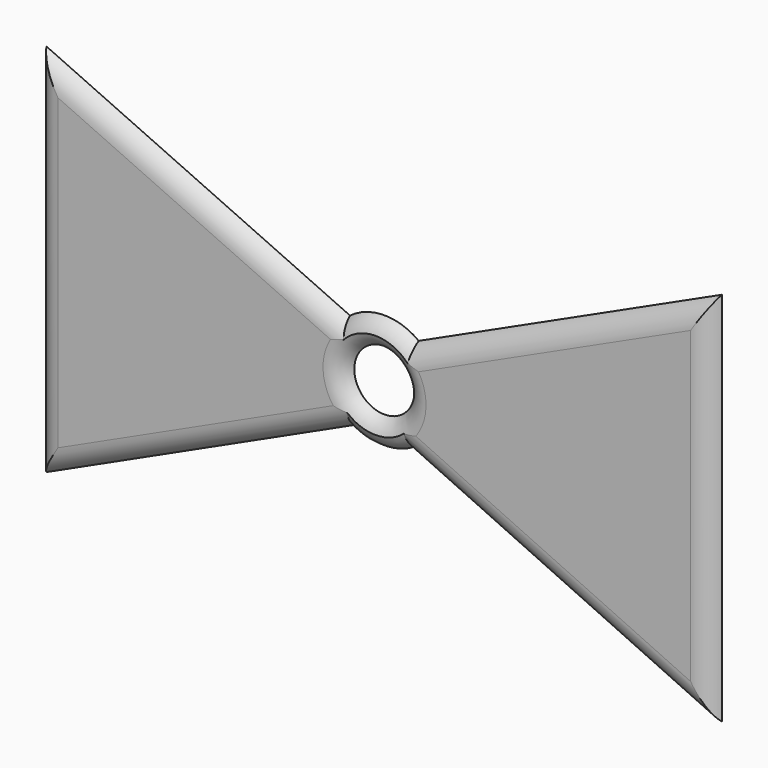
from build123d import *

# Parameters (mm, degrees)
F1_DEPTH     = 2.54
F2_T1_DEPTH  = 99.1010776341
F2_T3_DEPTH  = 99.3158813996
F2_T8_DEPTH  = 90.6208911446
F2_S9_R      = 11.7840069811
F2_T10_DEPTH = 49
F2_T14_DEPTH = 91.7966915257
F2_S15_R     = 11.7840069811
F2_T16_DEPTH = 49
F2_T20_ANGLE = 169.5184876271
F2_T26_ANGLE = 180.7013968541
F2_T32_DEPTH = 90.6339735213
F2_S33_R     = 11.7840069811
F2_T34_DEPTH = 49
F2_T38_DEPTH = 91.7098992775
F2_S39_R     = 11.7840069811
F2_T40_DEPTH = 49
F2_T47_DEPTH = 90.6208911446
F2_S48_R     = 11.7840069811
F2_T49_DEPTH = 49
F2_T52_ANGLE = 180.7013968541
F2_T60_DEPTH = 91.7966915257
F2_S61_R     = 11.7840069811
F2_T62_DEPTH = 49
F2_T65_ANGLE = 169.5184876271
F2_T73_ANGLE = 169.5184876271
F2_T78_DEPTH = 91.7098992775
F2_S79_R     = 11.7840069811
F2_T80_DEPTH = 49
F2_T86_DEPTH = 90.6339735213
F2_S87_R     = 11.7840069811
F2_T88_DEPTH = 49
F2_T91_ANGLE = 180.7013968541


# Not quite as in the source:
# - a fillet or chamfer that OpenCascade refuses, or shapes differently, is made with other operations: its cross-section is extruded or revolved along the edge and cut away or added


with BuildPart() as f1:
    # F0 (on Front) → F1 (new body)
    with BuildSketch(Plane.XZ):
        with BuildLine():
            Line((-31.3936966788, 53.9309575686), (-93.8453510125, 82.3742888697))
            Line((-93.8453510125, 82.3742888697), (-93.8453510125, 5.2702564917))
            Line((-93.8453510125, 5.2702564917), (-30.4330390113, 34.4399206311))
            ThreePointArc((-30.4330390113, 34.4399206311), (-36.0837561517, 43.9306053941), (-31.3936966788, 53.9309575686))
        make_face()
        with BuildLine():
            Line((-24.3140361377, 37.2546620127), (-30.4330390113, 34.4399206311))
            ThreePointArc((-30.4330390113, 34.4399206311), (-24.3162174043, 32.7266945746), (-18.1987619666, 34.4376560178))
            Line((-18.1987619666, 34.4376560178), (-24.3140361377, 37.2546620127))
        make_face()
        with BuildLine():
            ThreePointArc((-17.2562665131, 53.9473696458), (-24.3277161277, 56.2947003943), (-31.3936966788, 53.9309575686))
            Line((-31.3936966788, 53.9309575686), (-24.3140361377, 50.7065573118))
            Line((-24.3140361377, 50.7065573118), (-17.2562665131, 53.9473696458))
        make_face()
        with BuildLine():
            Line((-24.3140361377, 50.7065573118), (-31.3936966788, 53.9309575686))
            ThreePointArc((-31.3936966788, 53.9309575686), (-36.0837561517, 43.9306053941), (-30.4330390113, 34.4399206311))
            Line((-30.4330390113, 34.4399206311), (-24.3140361377, 37.2546620127))
            Line((-24.3140361377, 37.2546620127), (-18.1987619666, 34.4376560178))
            ThreePointArc((-18.1987619666, 34.4376560178), (-14.0445362947, 38.731411302), (-12.5300291567, 44.5107013538))
            ThreePointArc((-12.5300291567, 44.5107013538), (-13.7776319348, 49.7877276945), (-17.2562665131, 53.9473696458))
            Line((-17.2562665131, 53.9473696458), (-24.3140361377, 50.7065573118))
        make_face()
        with BuildLine():
            ThreePointArc((-18.1181801797, 44.5107013538), (-28.6951679009, 40.1295695906), (-24.3140361377, 50.7065573118))
            ThreePointArc((-24.3140361377, 50.7065573118), (-19.9329043745, 48.891833117), (-18.1181801797, 44.5107013538))
        make_face(mode=Mode.SUBTRACT)
        with BuildLine():
            Line((45.1190461185, 82.5890926352), (-17.2562665131, 53.9473696458))
            ThreePointArc((-17.2562665131, 53.9473696458), (-13.7776319348, 49.7877276945), (-12.5300291567, 44.5107013538))
            ThreePointArc((-12.5300291567, 44.5107013538), (-14.0445362947, 38.731411302), (-18.1987619666, 34.4376560178))
            Line((-18.1987619666, 34.4376560178), (45.1190461185, 5.2702564917))
            Line((45.1190461185, 5.2702564917), (45.1190461185, 82.5890926352))
        make_face()
    extrude(amount=F1_DEPTH)

    # F2: fillet of radius 5.08 on 9 edges, made by hand

    # F2_s2 → F2_t1 (cut)
    with BuildSketch(Plane.XY.offset(-5.7282661364)):
        with BuildLine():
            ThreePointArc((-93.8453510125, 0), (-91.9859419613, -1.8594090512), (-89.4459419613, -2.54))
            Line((-89.4459419613, -2.54), (-89.4459419613, -2.6416))
            Line((-89.4459419613, -2.6416), (-93.8453510125, -2.6416))
            Line((-93.8453510125, -2.6416), (-93.9469510125, -2.54))
            ThreePointArc((-93.9469510125, -2.54), (-93.9469510125, -1.27), (-93.9333391936, -0.0508))
            Line((-93.9333391936, -0.0508), (-93.8453510125, 0))
        make_face()
    extrude(amount=F2_T1_DEPTH, mode=Mode.SUBTRACT)

    # F2_s4 → F2_t3 (cut)
    with BuildSketch(Plane.XY.offset(-5.7282661364)):
        with BuildLine():
            ThreePointArc((45.1190461184, 0), (43.2596370672, -1.8594090512), (40.7196370672, -2.54))
            Line((40.7196370672, -2.54), (40.7196370672, -2.6416))
            Line((40.7196370672, -2.6416), (45.1190461185, -2.6416))
            Line((45.1190461185, -2.6416), (45.2206461185, -2.54))
            ThreePointArc((45.2206461185, -2.54), (45.2206461185, -1.27), (45.2070342995, -0.0508))
            Line((45.2070342995, -0.0508), (45.1190461184, 0))
        make_face()
    extrude(amount=F2_T3_DEPTH, mode=Mode.SUBTRACT)


with BuildPart() as f2_tool6:
    # F2_s7 → F2_t8 (new body)
    with BuildSketch(Plane(origin=(-36.3340032464, 0, 16.54816198), x_dir=(0, 1, 0), z_dir=(-0.9100576268, 0, 0.4144817437))):
        with BuildLine():
            ThreePointArc((0, -36.0681651183), (-1.8594090512, -34.2087560671), (-2.54, -31.6687560671))
            Line((-2.54, -31.6687560671), (-2.6416, -31.6687560671))
            Line((-2.6416, -31.6687560671), (-2.6416, -36.0681651183))
            Line((-2.6416, -36.0681651183), (-2.54, -36.1697651183))
            ThreePointArc((-2.54, -36.1697651183), (-1.27, -36.1697651183), (-0.0508, -36.1561532993))
            Line((-0.0508, -36.1561532993), (0, -36.0681651183))
        make_face()
    extrude(amount=F2_T8_DEPTH)

    # F2_s9 → F2_t10 (cut, symmetric)
    with BuildSketch(Plane.XZ.offset(1.3)):
        with Locations((-24.3140361377, 44.5107013538)):
            Circle(F2_S9_R)
    extrude(amount=F2_T10_DEPTH, both=True, mode=Mode.SUBTRACT)


with BuildPart() as f1_1:
    add(f1.part)

    # F2_t5: cut F2_tool6
    add(f2_tool6.part, mode=Mode.SUBTRACT)


with BuildPart() as f2_tool12:
    # F2_s13 → F2_t14 (new body)
    with BuildSketch(Plane(origin=(-85.4468499724, 0, -39.3055518212), x_dir=(0, 1, 0), z_dir=(0.9084904493, 0, 0.4179056155))):
        with BuildLine():
            ThreePointArc((0, 44.0064768695), (-1.8594090512, 45.8658859207), (-2.54, 48.4058859207))
            Line((-2.54, 48.4058859207), (-2.6416, 48.4058859207))
            Line((-2.6416, 48.4058859207), (-2.6416, 44.0064768695))
            Line((-2.6416, 44.0064768695), (-2.54, 43.9048768695))
            ThreePointArc((-2.54, 43.9048768695), (-1.27, 43.9048768695), (-0.0508, 43.9184886885))
            Line((-0.0508, 43.9184886885), (0, 44.0064768695))
        make_face()
    extrude(amount=F2_T14_DEPTH)

    # F2_s15 → F2_t16 (cut, symmetric)
    with BuildSketch(Plane.XZ.offset(1.3)):
        with Locations((-24.3140361377, 44.5107013538)):
            Circle(F2_S15_R)
    extrude(amount=F2_T16_DEPTH, both=True, mode=Mode.SUBTRACT)


with BuildPart() as f1_2:
    add(f1_1.part)

    # F2_t11: cut F2_tool12
    add(f2_tool12.part, mode=Mode.SUBTRACT)


with BuildPart() as f2_tool18:
    # F2_s19 → F2_t20 (revolve)
    with BuildSketch(Plane(origin=(-4.2425907564, 0, 46.3479960774), x_dir=(0, 1, 0), z_dir=(-0.0911566276, 0, 0.9958365675))):
        with BuildLine():
            ThreePointArc((0, 31.939367846), (-1.8594090512, 30.0799587948), (-2.54, 27.5399587948))
            Line((-2.54, 27.5399587948), (-2.6416, 27.5399587948))
            Line((-2.6416, 27.5399587948), (-2.6416, 31.939367846))
            Line((-2.6416, 31.939367846), (-2.54, 32.040967846))
            ThreePointArc((-2.54, 32.040967846), (-1.27, 32.040967846), (-0.0508, 32.027356027))
            Line((-0.0508, 32.027356027), (0, 31.939367846))
        make_face()
    revolve(axis=Axis((-24.3140361377, -2.54, 44.5107013538), (0, -1, 0)), revolution_arc=F2_T20_ANGLE)

    split(bisect_by=Plane(origin=(-18.3905538043, 0, 39.9794639438), x_dir=(0, 1, 0), z_dir=(0.4179056155, 0, -0.9084904493)), keep=Keep.TOP)

    split(bisect_by=Plane(origin=(9.9009901007, 0, 21.4934824919), x_dir=(0, 1, 0), z_dir=(-0.4183934216, 0, -0.9082658998)), keep=Keep.TOP)


with BuildPart() as f1_3:
    add(f1_2.part)

    # F2_t17: cut F2_tool18
    add(f2_tool18.part, mode=Mode.SUBTRACT)


with BuildPart() as f2_tool24:
    # F2_s25 → F2_t26 (revolve)
    with BuildSketch(Plane(origin=(0.2201689694, 0, 44.3890119894), x_dir=(0, 1, 0), z_dir=(-0.004959927, 0, -0.9999876995))):
        with BuildLine():
            ThreePointArc((0, -12.7504999131), (-1.8594090512, -14.6099089643), (-2.54, -17.1499089643))
            Line((-2.54, -17.1499089643), (-2.6416, -17.1499089643))
            Line((-2.6416, -17.1499089643), (-2.6416, -12.7504999131))
            Line((-2.6416, -12.7504999131), (-2.54, -12.6488999131))
            ThreePointArc((-2.54, -12.6488999131), (-1.27, -12.6488999131), (-0.0508, -12.6625117321))
            Line((-0.0508, -12.6625117321), (0, -12.7504999131))
        make_face()
    revolve(axis=Axis((-24.3140361377, -2.54, 44.5107013538), (0, -1, 0)), revolution_arc=F2_T26_ANGLE)

    split(bisect_by=Plane(origin=(14.9495959692, 0, 32.824108752), x_dir=(0, 1, 0), z_dir=(0.4144817437, 0, 0.9100576268)), keep=Keep.TOP)

    split(bisect_by=Plane(origin=(-23.4630512937, 0, 51.0973156286), x_dir=(0, 1, 0), z_dir=(-0.4172931935, 0, 0.9087719134)), keep=Keep.TOP)


with BuildPart() as f1_4:
    add(f1_3.part)

    # F2_t23: cut F2_tool24
    add(f2_tool24.part, mode=Mode.SUBTRACT)


with BuildPart() as f2_tool30:
    # F2_s31 → F2_t32 (new body)
    with BuildSketch(Plane(origin=(78.5772458658, 0, 36.0813856381), x_dir=(0, 1, 0), z_dir=(-0.9087719134, 0, -0.4172931935))):
        with BuildLine():
            ThreePointArc((0, -56.2267768991), (-1.8594090512, -54.3673678478), (-2.54, -51.8273678478))
            Line((-2.54, -51.8273678478), (-2.6416, -51.8273678478))
            Line((-2.6416, -51.8273678478), (-2.6416, -56.2267768991))
            Line((-2.6416, -56.2267768991), (-2.54, -56.3283768991))
            ThreePointArc((-2.54, -56.3283768991), (-1.27, -56.3283768991), (-0.0508, -56.3147650801))
            Line((-0.0508, -56.3147650801), (0, -56.2267768991))
        make_face()
    extrude(amount=F2_T32_DEPTH)

    # F2_s33 → F2_t34 (cut, symmetric)
    with BuildSketch(Plane.XZ.offset(1.3)):
        with Locations((-24.3140361377, 44.5107013538)):
            Circle(F2_S33_R)
    extrude(amount=F2_T34_DEPTH, both=True, mode=Mode.SUBTRACT)


with BuildPart() as f1_5:
    add(f1_4.part)

    # F2_t29: cut F2_tool30
    add(f2_tool30.part, mode=Mode.SUBTRACT)


with BuildPart() as f2_tool36:
    # F2_s37 → F2_t38 (new body)
    with BuildSketch(Plane(origin=(-38.0893351185, 0, 17.5458830412), x_dir=(0, 1, 0), z_dir=(0.9082658998, 0, -0.4183934216))):
        with BuildLine():
            ThreePointArc((0, 23.6643063411), (-1.8594090512, 25.5237153923), (-2.54, 28.0637153923))
            Line((-2.54, 28.0637153923), (-2.6416, 28.0637153923))
            Line((-2.6416, 28.0637153923), (-2.6416, 23.6643063411))
            Line((-2.6416, 23.6643063411), (-2.54, 23.5627063411))
            ThreePointArc((-2.54, 23.5627063411), (-1.27, 23.5627063411), (-0.0508, 23.57631816))
            Line((-0.0508, 23.57631816), (0, 23.6643063411))
        make_face()
    extrude(amount=F2_T38_DEPTH)

    # F2_s39 → F2_t40 (cut, symmetric)
    with BuildSketch(Plane.XZ.offset(1.3)):
        with Locations((-24.3140361377, 44.5107013538)):
            Circle(F2_S39_R)
    extrude(amount=F2_T40_DEPTH, both=True, mode=Mode.SUBTRACT)


with BuildPart() as f1_6:
    add(f1_5.part)

    # F2_t35: cut F2_tool36
    add(f2_tool36.part, mode=Mode.SUBTRACT)

    # F2_s41 → F2_t42 (revolve, cut)
    with BuildSketch(Plane.YZ.offset(-24.3140361377)):
        with BuildLine():
            ThreePointArc((0, 50.7065573118), (-1.8594090512, 52.565966363), (-2.54, 55.105966363))
            Line((-2.54, 55.105966363), (-2.6416, 55.105966363))
            Line((-2.6416, 55.105966363), (-2.6416, 50.7065573118))
            Line((-2.6416, 50.7065573118), (-2.54, 50.6049573118))
            ThreePointArc((-2.54, 50.6049573118), (-1.27, 50.6049573118), (-0.0508, 50.6185691308))
            Line((-0.0508, 50.6185691308), (0, 50.7065573118))
        make_face()
    revolve(axis=Axis((-24.3140361377, -2.54, 44.5107013538), (0, 1, 0)), mode=Mode.SUBTRACT)


with BuildPart() as f2_tool45:
    # F2_s46 → F2_t47 (new body)
    with BuildSketch(Plane(origin=(-36.3340032464, 0, 16.54816198), x_dir=(0, 1, 0), z_dir=(-0.9100576268, 0, 0.4144817437))):
        with BuildLine():
            ThreePointArc((0, -36.0681651183), (-1.8594090512, -34.2087560671), (-2.54, -31.6687560671))
            Line((-2.54, -31.6687560671), (-2.6416, -31.6687560671))
            Line((-2.6416, -31.6687560671), (-2.6416, -36.0681651183))
            Line((-2.6416, -36.0681651183), (-2.54, -36.1697651183))
            ThreePointArc((-2.54, -36.1697651183), (-1.27, -36.1697651183), (-0.0508, -36.1561532993))
            Line((-0.0508, -36.1561532993), (0, -36.0681651183))
        make_face()
    extrude(amount=F2_T47_DEPTH)

    # F2_s48 → F2_t49 (intersect, symmetric)
    with BuildSketch(Plane.XZ.offset(1.3)):
        with Locations((-24.3140361377, 44.5107013538)):
            Circle(F2_S48_R)
    extrude(amount=F2_T49_DEPTH, both=True, mode=Mode.INTERSECT)


with BuildPart() as f2_tool50:
    # F2_s51 → F2_t52 (revolve)
    with BuildSketch(Plane(origin=(0.2201689694, 0, 44.3890119894), x_dir=(0, 1, 0), z_dir=(-0.004959927, 0, -0.9999876995))):
        with BuildLine():
            ThreePointArc((0, -12.7504999131), (-1.8594090512, -14.6099089643), (-2.54, -17.1499089643))
            Line((-2.54, -17.1499089643), (-2.6416, -17.1499089643))
            Line((-2.6416, -17.1499089643), (-2.6416, -12.7504999131))
            Line((-2.6416, -12.7504999131), (-2.54, -12.6488999131))
            ThreePointArc((-2.54, -12.6488999131), (-1.27, -12.6488999131), (-0.0508, -12.6625117321))
            Line((-0.0508, -12.6625117321), (0, -12.7504999131))
        make_face()
    revolve(axis=Axis((-24.3140361377, -2.54, 44.5107013538), (0, -1, 0)), revolution_arc=F2_T52_ANGLE)

    split(bisect_by=Plane(origin=(14.9495959692, 0, 32.824108752), x_dir=(0, 1, 0), z_dir=(-0.4144817437, 0, -0.9100576268)), keep=Keep.TOP)

    split(bisect_by=Plane(origin=(-23.4630512937, 0, 51.0973156286), x_dir=(0, 1, 0), z_dir=(-0.4172931935, 0, 0.9087719134)), keep=Keep.TOP)


with BuildPart() as f2_tool45_1:
    add(f2_tool45.part)

    # F2_t55: intersect F2_tool50
    add(f2_tool50.part, mode=Mode.INTERSECT)


with BuildPart() as f1_7:
    add(f1_6.part)

    # F2_t43: cut F2_tool45
    add(f2_tool45_1.part, mode=Mode.SUBTRACT)


with BuildPart() as f2_tool58:
    # F2_s59 → F2_t60 (new body)
    with BuildSketch(Plane(origin=(-85.4468499724, 0, -39.3055518212), x_dir=(0, 1, 0), z_dir=(0.9084904493, 0, 0.4179056155))):
        with BuildLine():
            ThreePointArc((0, 44.0064768695), (-1.8594090512, 45.8658859207), (-2.54, 48.4058859207))
            Line((-2.54, 48.4058859207), (-2.6416, 48.4058859207))
            Line((-2.6416, 48.4058859207), (-2.6416, 44.0064768695))
            Line((-2.6416, 44.0064768695), (-2.54, 43.9048768695))
            ThreePointArc((-2.54, 43.9048768695), (-1.27, 43.9048768695), (-0.0508, 43.9184886885))
            Line((-0.0508, 43.9184886885), (0, 44.0064768695))
        make_face()
    extrude(amount=F2_T60_DEPTH)

    # F2_s61 → F2_t62 (intersect, symmetric)
    with BuildSketch(Plane.XZ.offset(1.3)):
        with Locations((-24.3140361377, 44.5107013538)):
            Circle(F2_S61_R)
    extrude(amount=F2_T62_DEPTH, both=True, mode=Mode.INTERSECT)


with BuildPart() as f2_tool63:
    # F2_s64 → F2_t65 (revolve)
    with BuildSketch(Plane(origin=(-4.2425907564, 0, 46.3479960774), x_dir=(0, 1, 0), z_dir=(-0.0911566276, 0, 0.9958365675))):
        with BuildLine():
            ThreePointArc((0, 31.939367846), (-1.8594090512, 30.0799587948), (-2.54, 27.5399587948))
            Line((-2.54, 27.5399587948), (-2.6416, 27.5399587948))
            Line((-2.6416, 27.5399587948), (-2.6416, 31.939367846))
            Line((-2.6416, 31.939367846), (-2.54, 32.040967846))
            ThreePointArc((-2.54, 32.040967846), (-1.27, 32.040967846), (-0.0508, 32.027356027))
            Line((-0.0508, 32.027356027), (0, 31.939367846))
        make_face()
    revolve(axis=Axis((-24.3140361377, -2.54, 44.5107013538), (0, -1, 0)), revolution_arc=F2_T65_ANGLE)

    split(bisect_by=Plane(origin=(-18.3905538043, 0, 39.9794639438), x_dir=(0, 1, 0), z_dir=(-0.4179056155, 0, 0.9084904493)), keep=Keep.TOP)

    split(bisect_by=Plane(origin=(9.9009901007, 0, 21.4934824919), x_dir=(0, 1, 0), z_dir=(-0.4183934216, 0, -0.9082658998)), keep=Keep.TOP)


with BuildPart() as f2_tool58_1:
    add(f2_tool58.part)

    # F2_t68: intersect F2_tool63
    add(f2_tool63.part, mode=Mode.INTERSECT)


with BuildPart() as f1_8:
    add(f1_7.part)

    # F2_t56: cut F2_tool58
    add(f2_tool58_1.part, mode=Mode.SUBTRACT)


with BuildPart() as f2_tool71:
    # F2_s72 → F2_t73 (revolve)
    with BuildSketch(Plane(origin=(-4.2425907564, 0, 46.3479960774), x_dir=(0, 1, 0), z_dir=(-0.0911566276, 0, 0.9958365675))):
        with BuildLine():
            ThreePointArc((0, 31.939367846), (-1.8594090512, 30.0799587948), (-2.54, 27.5399587948))
            Line((-2.54, 27.5399587948), (-2.6416, 27.5399587948))
            Line((-2.6416, 27.5399587948), (-2.6416, 31.939367846))
            Line((-2.6416, 31.939367846), (-2.54, 32.040967846))
            ThreePointArc((-2.54, 32.040967846), (-1.27, 32.040967846), (-0.0508, 32.027356027))
            Line((-0.0508, 32.027356027), (0, 31.939367846))
        make_face()
    revolve(axis=Axis((-24.3140361377, -2.54, 44.5107013538), (0, -1, 0)), revolution_arc=F2_T73_ANGLE)

    split(bisect_by=Plane(origin=(-18.3905538043, 0, 39.9794639438), x_dir=(0, 1, 0), z_dir=(0.4179056155, 0, -0.9084904493)), keep=Keep.TOP)

    split(bisect_by=Plane(origin=(9.9009901007, 0, 21.4934824919), x_dir=(0, 1, 0), z_dir=(0.4183934216, 0, 0.9082658998)), keep=Keep.TOP)


with BuildPart() as f2_tool76:
    # F2_s77 → F2_t78 (new body)
    with BuildSketch(Plane(origin=(-38.0893351185, 0, 17.5458830412), x_dir=(0, 1, 0), z_dir=(0.9082658998, 0, -0.4183934216))):
        with BuildLine():
            ThreePointArc((0, 23.6643063411), (-1.8594090512, 25.5237153923), (-2.54, 28.0637153923))
            Line((-2.54, 28.0637153923), (-2.6416, 28.0637153923))
            Line((-2.6416, 28.0637153923), (-2.6416, 23.6643063411))
            Line((-2.6416, 23.6643063411), (-2.54, 23.5627063411))
            ThreePointArc((-2.54, 23.5627063411), (-1.27, 23.5627063411), (-0.0508, 23.57631816))
            Line((-0.0508, 23.57631816), (0, 23.6643063411))
        make_face()
    extrude(amount=F2_T78_DEPTH)

    # F2_s79 → F2_t80 (intersect, symmetric)
    with BuildSketch(Plane.XZ.offset(1.3)):
        with Locations((-24.3140361377, 44.5107013538)):
            Circle(F2_S79_R)
    extrude(amount=F2_T80_DEPTH, both=True, mode=Mode.INTERSECT)


with BuildPart() as f2_tool71_1:
    add(f2_tool71.part)

    # F2_t81: intersect F2_tool76
    add(f2_tool76.part, mode=Mode.INTERSECT)


with BuildPart() as f1_9:
    add(f1_8.part)

    # F2_t69: cut F2_tool71
    add(f2_tool71_1.part, mode=Mode.SUBTRACT)


with BuildPart() as f2_tool84:
    # F2_s85 → F2_t86 (new body)
    with BuildSketch(Plane(origin=(78.5772458658, 0, 36.0813856381), x_dir=(0, 1, 0), z_dir=(-0.9087719134, 0, -0.4172931935))):
        with BuildLine():
            ThreePointArc((0, -56.2267768991), (-1.8594090512, -54.3673678478), (-2.54, -51.8273678478))
            Line((-2.54, -51.8273678478), (-2.6416, -51.8273678478))
            Line((-2.6416, -51.8273678478), (-2.6416, -56.2267768991))
            Line((-2.6416, -56.2267768991), (-2.54, -56.3283768991))
            ThreePointArc((-2.54, -56.3283768991), (-1.27, -56.3283768991), (-0.0508, -56.3147650801))
            Line((-0.0508, -56.3147650801), (0, -56.2267768991))
        make_face()
    extrude(amount=F2_T86_DEPTH)

    # F2_s87 → F2_t88 (intersect, symmetric)
    with BuildSketch(Plane.XZ.offset(1.3)):
        with Locations((-24.3140361377, 44.5107013538)):
            Circle(F2_S87_R)
    extrude(amount=F2_T88_DEPTH, both=True, mode=Mode.INTERSECT)


with BuildPart() as f2_tool89:
    # F2_s90 → F2_t91 (revolve)
    with BuildSketch(Plane(origin=(0.2201689694, 0, 44.3890119894), x_dir=(0, 1, 0), z_dir=(-0.004959927, 0, -0.9999876995))):
        with BuildLine():
            ThreePointArc((0, -12.7504999131), (-1.8594090512, -14.6099089643), (-2.54, -17.1499089643))
            Line((-2.54, -17.1499089643), (-2.6416, -17.1499089643))
            Line((-2.6416, -17.1499089643), (-2.6416, -12.7504999131))
            Line((-2.6416, -12.7504999131), (-2.54, -12.6488999131))
            ThreePointArc((-2.54, -12.6488999131), (-1.27, -12.6488999131), (-0.0508, -12.6625117321))
            Line((-0.0508, -12.6625117321), (0, -12.7504999131))
        make_face()
    revolve(axis=Axis((-24.3140361377, -2.54, 44.5107013538), (0, -1, 0)), revolution_arc=F2_T91_ANGLE)

    split(bisect_by=Plane(origin=(14.9495959692, 0, 32.824108752), x_dir=(0, 1, 0), z_dir=(0.4144817437, 0, 0.9100576268)), keep=Keep.TOP)

    split(bisect_by=Plane(origin=(-23.4630512937, 0, 51.0973156286), x_dir=(0, 1, 0), z_dir=(0.4172931935, 0, -0.9087719134)), keep=Keep.TOP)


with BuildPart() as f2_tool84_1:
    add(f2_tool84.part)

    # F2_t94: intersect F2_tool89
    add(f2_tool89.part, mode=Mode.INTERSECT)


with BuildPart() as f1_10:
    add(f1_9.part)

    # F2_t82: cut F2_tool84
    add(f2_tool84_1.part, mode=Mode.SUBTRACT)


solid = f1_10.part
